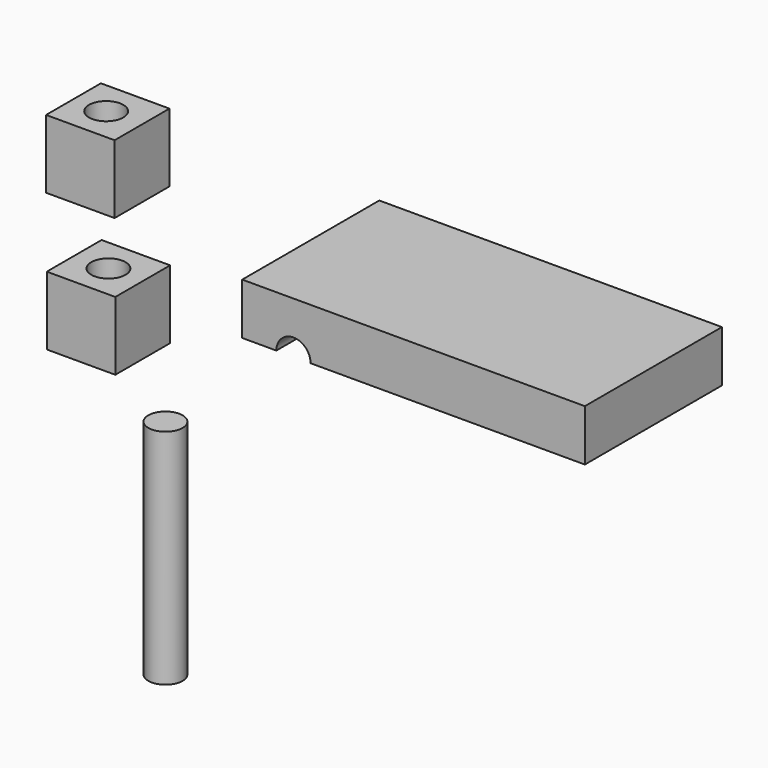
from build123d import *

# Parameters (mm, degrees)
F1_W      = 127
F1_H      = 63.5
F2_DEPTH  = 19.05
F3_R      = 6.35
F4_DEPTH  = 88.392
F0_R      = 6.35
F5_DEPTH  = 39.116
F6_DEPTH  = 43.434
F7_W      = 25.4
F7_H      = 25.4
F8_DEPTH  = 25.4
F10_DEPTH = 25.4
F11_R     = 6.35
F12_DEPTH = 47.244
F9_R      = 6.35
F13_DEPTH = 46.99


# Not quite as in the source:
# - a feature names something its author has since deleted; it is built from what else it names


with BuildPart() as f2:
    # F1 (on Top) → F2 (new body)
    with BuildSketch(Plane.XY):
        with Locations((44.5008012414, 28.5242010134)):
            Rectangle(F1_W, F1_H)
    extrude(amount=F2_DEPTH)

    # F3 (on face) → F4 (cut)
    with BuildSketch(Plane.XZ.offset(3.2257989866)):
        Circle(F3_R)
    extrude(amount=-F4_DEPTH, mode=Mode.SUBTRACT)


with BuildPart() as f5:
    # F0 (on Top) → F5 (new body)
    with BuildSketch(Plane.XY):
        with Locations((43.3363690972, -116.7080551386)):
            Circle(F0_R)
    extrude(amount=F5_DEPTH)

    # F6 (add): a face of the model
    f6_faces = [f5.faces().sort_by_distance(p)[0] for p in [
        (43.3363690972, -116.7080551386, 0),
    ]]
    extrude(f6_faces, amount=F6_DEPTH)


with BuildPart() as f8:
    # F7 (on Front) → F8 (new body)
    with BuildSketch(Plane.XZ):
        with Locations((-61.2544928074, 51.2233350098)):
            Rectangle(F7_W, F7_H)
    extrude(amount=F8_DEPTH)

    # F9 (on face) → F13 (cut)
    with BuildSketch(Plane(origin=(0, 0, 38.5233350098), x_dir=(1, 0, 0), z_dir=(0, 0, -1))):
        with Locations((-61.8434809148, 12.7)):
            Circle(F9_R)
    extrude(amount=-F13_DEPTH, mode=Mode.SUBTRACT)


with BuildPart() as f10:
    # F7 (on Front) → F10 (new body)
    with BuildSketch(Plane.XZ):
        with Locations((-60.9968144774, 0.1707609415)):
            Rectangle(F7_W, F7_H)
    extrude(amount=F10_DEPTH)

    # F11 (on face) → F12 (cut)
    with BuildSketch(Plane(origin=(0, 0, -12.5292390585), x_dir=(1, 0, 0), z_dir=(0, 0, -1))):
        with Locations((-60.9968144774, 12.7)):
            Circle(F11_R)
    extrude(amount=-F12_DEPTH, mode=Mode.SUBTRACT)


solid = Compound([f2.part, f5.part, f8.part, f10.part])
